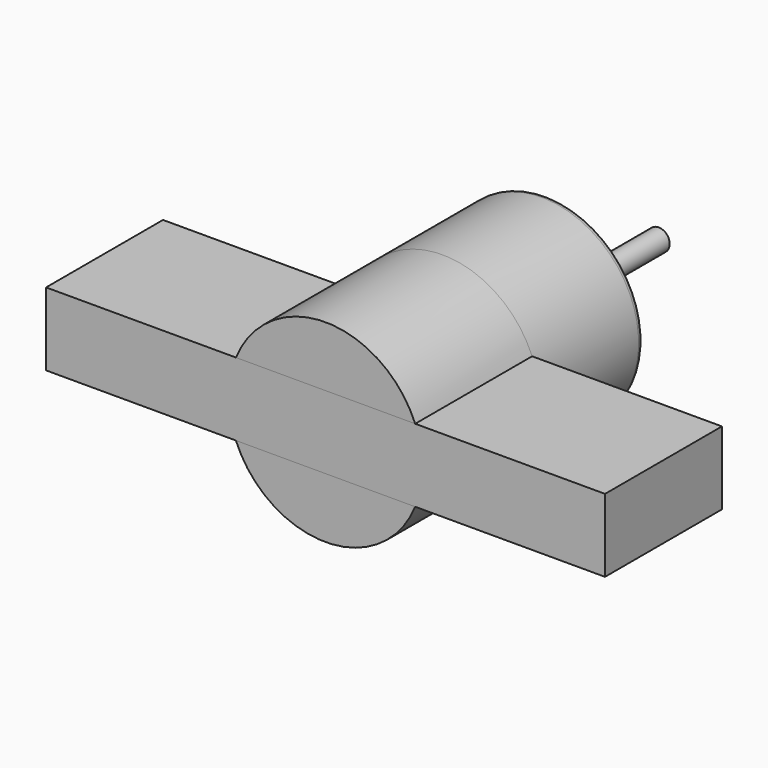
from build123d import *

# Parameters (mm, degrees)
F2_R     = 3
F4_DEPTH = 20
F5_DEPTH = 20


with BuildPart() as f1:
    # F0 (on Top) → F1 (revolve)
    with BuildSketch(Plane.XY):
        with BuildLine():
            Line((-13.25, 0), (0, 0))
            Line((0, 0), (0, 37))
            Line((0, 37), (-1.5, 37))
            Line((-1.5, 37), (-1.5, 16.6235913226))
            ThreePointArc((-1.5, 16.6235913226), (-6.4401709177, 12.3947665973), (-11.3803418353, 16.6235913226))
            Line((-11.3803418353, 16.6235913226), (-11.4607692348, 17.1388115494))
            ThreePointArc((-11.4607692348, 17.1388115494), (-12.4196143352, 17.8973036522), (-13.25, 17))
            Line((-13.25, 17), (-13.25, 0))
        make_face()
    revolve(axis=Axis((0, 18.5, 0), (0, -1, 0)))

    # F2
    f2_edges = [f1.edges().sort_by_distance(p)[0] for p in [
        (1.5, 16.623591, 0),
    ]]
    fillet(f2_edges, radius=F2_R)

    # F3 (on face) → F4 (join)
    with BuildSketch(Plane.XZ):
        with BuildLine():
            Line((-12.2703911918, 5), (-38.25, 5))
            Line((-38.25, 5), (-38.25, -5))
            Line((-38.25, -5), (-12.2703911918, -5))
            ThreePointArc((-12.2703911918, -5), (-13.25, 0), (-12.2703911918, 5))
        make_face()
        with BuildLine():
            Line((12.2703911918, 5), (-12.2703911918, 5))
            ThreePointArc((-12.2703911918, 5), (-13.25, 0), (-12.2703911918, -5))
            Line((-12.2703911918, -5), (12.2703911918, -5))
            ThreePointArc((12.2703911918, -5), (13.0027916866, -2.5475298535), (13.25, 0))
            ThreePointArc((13.25, 0), (13.0027916866, 2.5475298535), (12.2703911918, 5))
        make_face()
        with BuildLine():
            Line((38.25, 5), (12.2703911918, 5))
            ThreePointArc((12.2703911918, 5), (13.0027916866, 2.5475298535), (13.25, 0))
            ThreePointArc((13.25, 0), (13.0027916866, -2.5475298535), (12.2703911918, -5))
            Line((12.2703911918, -5), (38.25, -5))
            Line((38.25, -5), (38.25, 5))
        make_face()
    extrude(amount=F4_DEPTH)

    # F5 (add): faces of the model
    f5_faces = [f1.faces().sort_by_distance(p)[0] for p in [
        (0, 0, 8.4077666552),
        (0, 0, -8.4077666552),
    ]]
    extrude(f5_faces, amount=F5_DEPTH)


solid = f1.part
